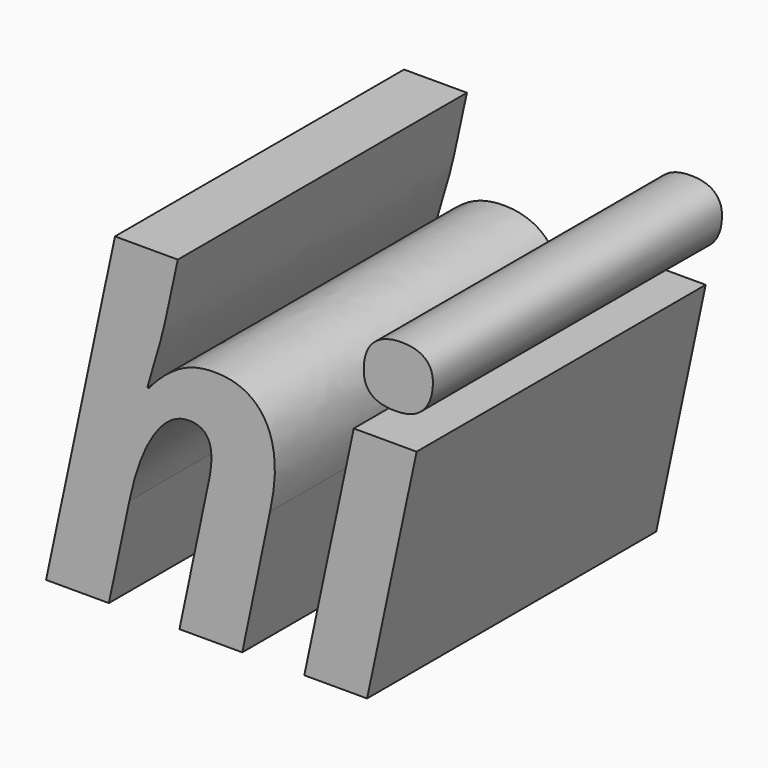
from build123d import *

# Parameters (mm, degrees)
F0_TEXT_SIZE = 30.0457287166
F1_DEPTH     = 25.4


# Not quite as in the source:
# - Text() gives the source's letters only with a copy of the font that has no kerning and outlines rounded to 1/6400 em; it was checked with that copy


with BuildPart() as f1:
    # F0 (on Front) → F1 (new body)
    with BuildSketch(Plane.XZ):
        with Locations((-35.6306955218, 24.0189060569)):
            Text('hi', F0_TEXT_SIZE, font='Open Sans', font_style=FontStyle.BOLDITALIC, text_align=(TextAlign.LEFT, TextAlign.BOTTOM))
    extrude(amount=F1_DEPTH)


solid = f1.part
